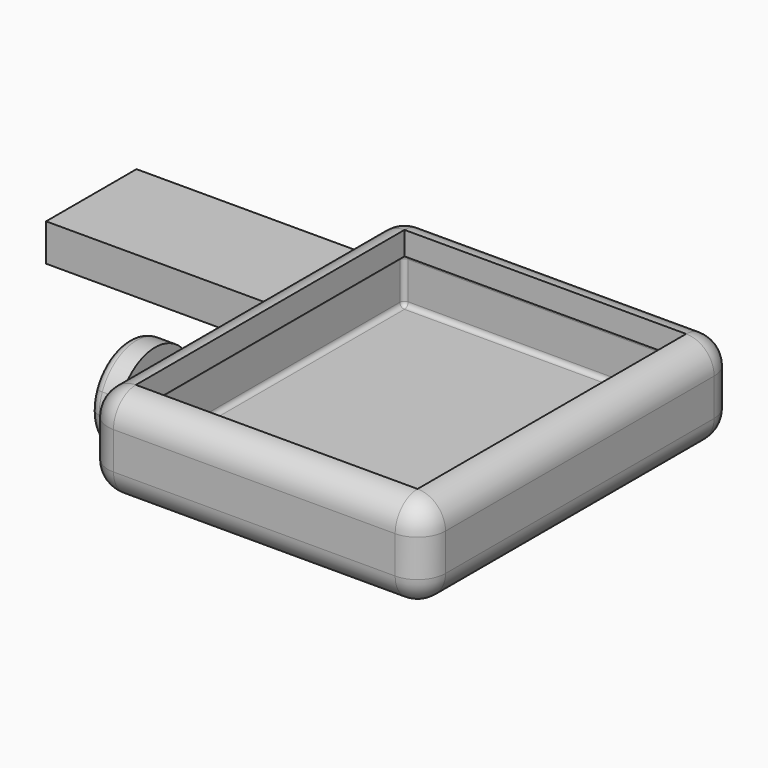
from build123d import *

# Parameters (mm, degrees)
F0_W     = 36.2
F0_H     = 42
F1_DEPTH = 10
F2_R     = 3
F3_T     = -2.5
F5_DEPTH = 3
F6_R     = 1
F7_W     = 12.1205560863
F7_H     = 4
F8_DEPTH = 25


# Not quite as in the source:
# - a shell that OpenCascade refuses in one call is made with other operations: the cavity is built on its own and cut out


with BuildPart() as f1:
    # F0 (on Top) → F1 (new body)
    with BuildSketch(Plane.XY):
        Rectangle(F0_W, F0_H)
    extrude(amount=F1_DEPTH)

    # F2
    f2_edges = [f1.edges().sort_by_distance(p)[0] for p in [
        (-18.1, -21, 5),
        (18.1, -21, 5),
        (0, -21, 0),
        (0, -21, 10),
        (-18.1, 21, 5),
        (-18.1, 0, 0),
        (-18.1, 0, 10),
        (18.1, 21, 5),
        (0, 21, 0),
        (0, 21, 10),
        (18.1, 0, 0),
        (18.1, 0, 10),
    ]]
    fillet(f2_edges, radius=F2_R)

    # F3: a shell. OpenCascade refuses it in one call, so the cavity is built on its own and cut out:
    # the body offset inwards by the wall thickness, plus a prism from it out through each open face.
    f3_core = offset(f1.part, amount=F3_T, mode=Mode.PRIVATE)
    f3_exits = [f3_core.faces().sort_by_distance(p)[0] for p in [
        (0, 0, 7.5),
    ]]
    add(f3_core, mode=Mode.SUBTRACT)
    extrude(f3_exits, amount=-F3_T, mode=Mode.SUBTRACT)

    # F4 (on face) → F5 (join)
    with BuildSketch(Plane(origin=(-18.1, 0, 0), x_dir=(0, -1, 0), z_dir=(-1, 0, 0))):
        with BuildLine():
            ThreePointArc((7.0906764033, 3), (11.6732520983, 0), (16.2558277932, 3))
            Line((16.2558277932, 3), (7.0906764033, 3))
        make_face()
        with BuildLine():
            Line((7.0906764033, 7), (16.2558277932, 7))
            ThreePointArc((16.2558277932, 7), (11.6732520983, 10), (7.0906764033, 7))
        make_face()
        with BuildLine():
            ThreePointArc((16.2558277932, 3), (16.5677836629, 3.9784517816), (16.6732520983, 5))
            ThreePointArc((16.6732520983, 5), (16.5677836629, 6.0215482184), (16.2558277932, 7))
            Line((16.2558277932, 7), (7.0906764033, 7))
            ThreePointArc((7.0906764033, 7), (6.6732520983, 5), (7.0906764033, 3))
            Line((7.0906764033, 3), (16.2558277932, 3))
        make_face()
    extrude(amount=F5_DEPTH)

    # F6
    f6_edges = [f1.edges().sort_by_distance(p)[0] for p in [
        (-21.1, -7.090676, 7),
    ]]
    fillet(f6_edges, radius=F6_R)

    # F7 (on face) → F8 (join)
    with BuildSketch(Plane(origin=(-18.1, 0, 0), x_dir=(0, -1, 0), z_dir=(-1, 0, 0))):
        with Locations((-11.0213514417, 5)):
            Rectangle(F7_W, F7_H)
    extrude(amount=F8_DEPTH)


solid = f1.part
